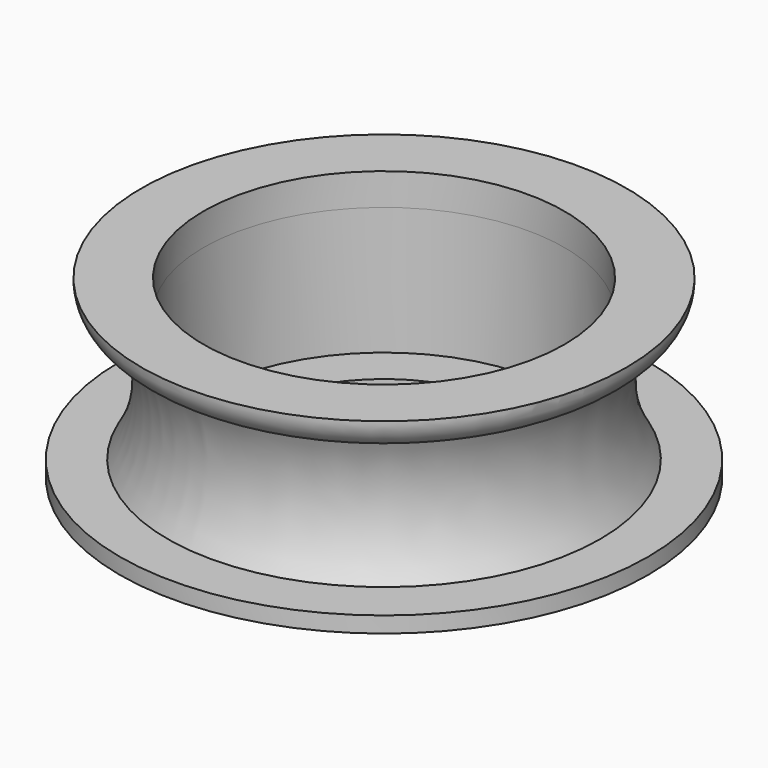
from build123d import *

# Parameters (mm, degrees)
F2_R     = 16.5358805208
F2_R_2   = 8.5
F3_DEPTH = 1
F4_R     = 15.1866700875
F4_R_2   = 11.3
F5_DEPTH = 2
F6_R     = 1.99999


# Not quite as in the source:
# - a fillet or chamfer is up to 0.001 mm smaller than in the source, because OpenCascade refuses the exact size


with BuildPart() as f1:
    # F0 (on Front) → F1 (revolve)
    with BuildSketch(Plane.XZ):
        with BuildLine():
            ThreePointArc((13.5358805208, -4), (12.3077325791, -0.0459885139), (13.1866700875, 4))
            Line((13.1866700875, 4), (11.3, 4))
            Line((11.3, 4), (11.3, -4))
            Line((11.3, -4), (13.5358805208, -4))
        make_face()
    revolve(axis=Axis((0, 0, -1.1675134301), (0, 0, -1)))

    # F2 (on face) → F3 (join)
    with BuildSketch(Plane(origin=(0, 0, -4), x_dir=(1, 0, 0), z_dir=(0, 0, -1))):
        Circle(F2_R)
        Circle(F2_R_2, mode=Mode.SUBTRACT)
    extrude(amount=F3_DEPTH)

    # F4 (on face) → F5 (join)
    with BuildSketch(Plane.XY.offset(4)):
        Circle(F4_R)
        Circle(F4_R_2, mode=Mode.SUBTRACT)
    extrude(amount=F5_DEPTH)

    # F6 (radius 2 in the source; OpenCascade refuses exactly that, so slightly less here)
    f6_edges = [f1.edges().sort_by_distance(p)[0] for p in [
        (-15.18667, 0, 4),
    ]]
    fillet(f6_edges, radius=F6_R)


solid = f1.part
